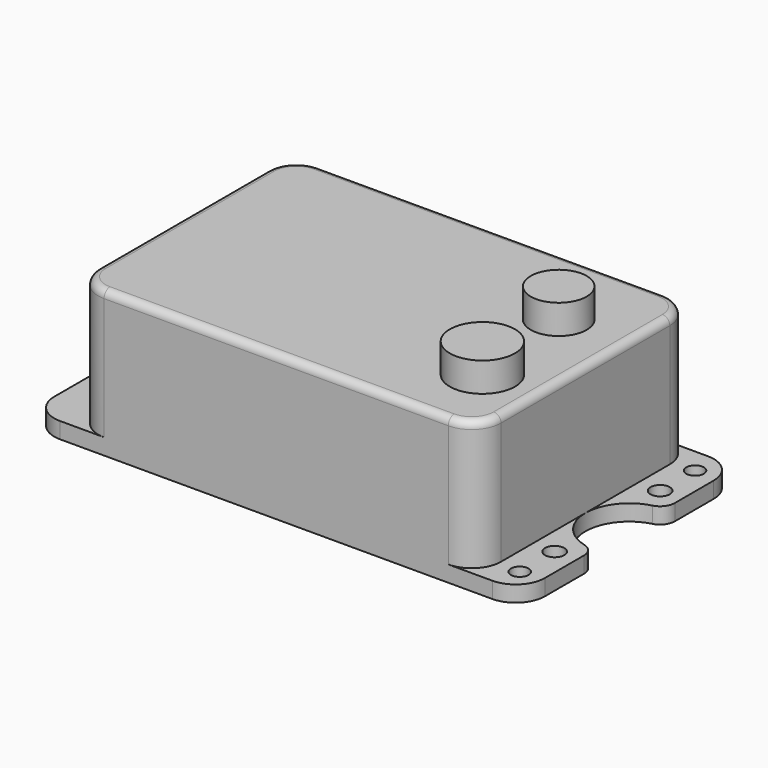
from build123d import *

# Parameters (mm, degrees)
F0_W      = 167.5
F0_H      = 92
F1_DEPTH  = 5.5
F2_W      = 137.5
F2_H      = 92
F3_DEPTH  = 49.7
F4_R      = 10
F5_R      = 2.54
F6_R      = 3.3
F6_R_2    = 3
F7_DEPTH  = 5.5
F10_DEPTH = 5.5
F11_R     = 5
F12_R     = 11.129920483
F12_R_2   = 9.5443004054
F13_DEPTH = 10


# Not quite as in the source:
# - a feature names something its author has since deleted; it is built from what else it names


with BuildPart() as f1:
    # F0 (on Top) → F1 (new body)
    with BuildSketch(Plane.XY):
        Rectangle(F0_W, F0_H)
    extrude(amount=F1_DEPTH)

    # F2 (on Top) → F3 (join)
    with BuildSketch(Plane.XY):
        Rectangle(F2_W, F2_H)
    extrude(amount=F3_DEPTH)

    # F4
    f4_edges = [f1.edges().sort_by_distance(p)[0] for p in [
        (-83.75, -46, 2.75),
        (83.75, -46, 2.75),
        (83.75, 46, 2.75),
        (-83.75, 46, 2.75),
        (-68.75, 46, 27.6),
        (-68.75, -46, 27.6),
        (68.75, 46, 27.6),
        (68.75, -46, 27.6),
    ]]
    fillet(f4_edges, radius=F4_R)

    # F5
    f5_edges = [f1.edges().sort_by_distance(p)[0] for p in [
        (0, -46, 49.7),
        (0, 46, 49.7),
        (65.821068, -43.071068, 49.7),
        (68.75, 0, 49.7),
        (65.821068, 43.071068, 49.7),
        (-65.821068, -43.071068, 49.7),
        (-68.75, 0, 49.7),
        (-65.821068, 43.071068, 49.7),
    ]]
    fillet(f5_edges, radius=F5_R)

    # F6 (on face) → F7 (cut)
    with BuildSketch(Plane.XY.offset(5.5)):
        with Locations((-76.25, 22.5)):
            Circle(F6_R)
        with Locations((-76.25, -22.5)):
            Circle(F6_R)
        with Locations((76.25, -22.5)):
            Circle(F6_R)
        with Locations((76.25, 22.5)):
            Circle(F6_R)
        with Locations((76.25, 37.4)):
            Circle(F6_R_2)
        with Locations((76.25, -37.4)):
            Circle(F6_R_2)
    extrude(amount=-F7_DEPTH, mode=Mode.SUBTRACT)

    # F8 (on face) + F9 (on face) → F10 (cut)
    with BuildSketch(Plane.XY.offset(5.5)):
        with BuildLine():
            ThreePointArc((-83.75, -15), (-73.1433982822, -10.6066017178), (-68.75, 0))
            ThreePointArc((-68.75, 0), (-73.1433982822, 10.6066017178), (-83.75, 15))
            Line((-83.75, 15), (-83.75, -15))
        make_face()
    with BuildSketch(Plane.XY.offset(5.5)):
        with BuildLine():
            Line((83.75, -15), (83.75, 15))
            ThreePointArc((83.75, 15), (73.1433983426, 10.6066017782), (68.75, 1.709e-07))
            ThreePointArc((68.75, 1.709e-07), (73.1433982218, -10.6066016574), (83.75, -15))
        make_face()
    extrude(amount=-F10_DEPTH, mode=Mode.SUBTRACT)

    # F11
    f11_edges = [f1.edges().sort_by_distance(p)[0] for p in [
        (83.75, -15, 2.75),
        (-83.75, -15, 2.75),
        (-83.75, 15, 2.75),
        (83.75, 15, 2.75),
    ]]
    fillet(f11_edges, radius=F11_R)

    # F12 (on face) → F13 (join)
    with BuildSketch(Plane.XY.offset(49.7)):
        with Locations((50.4262000322, -21.045640111)):
            Circle(F12_R)
        with Locations((46.4671105146, 16.4614468813)):
            Circle(F12_R_2)
    extrude(amount=F13_DEPTH)


solid = f1.part
